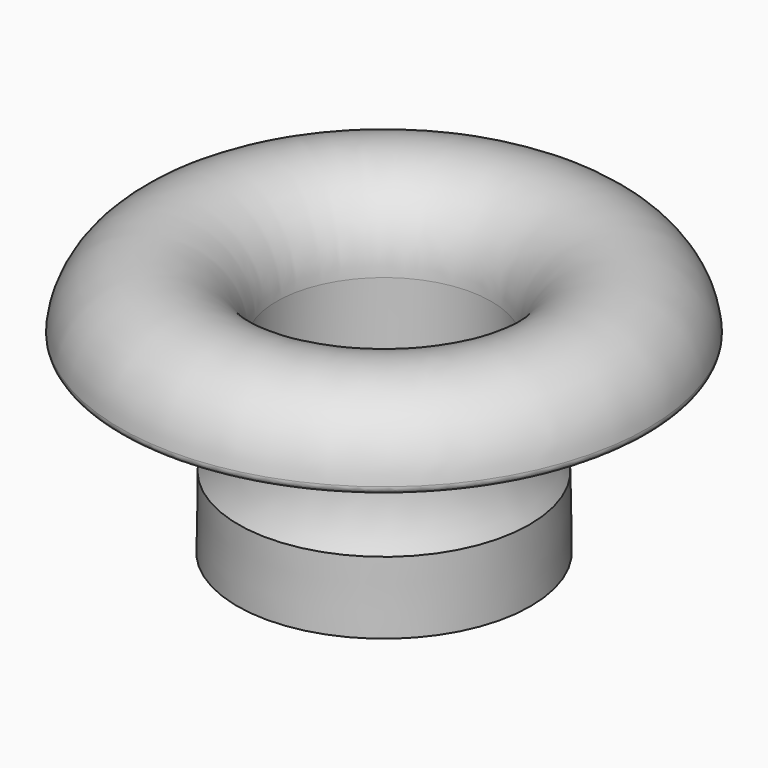
from build123d import *

# Parameters (mm, degrees)
F2_R    = 1
F3_SIZE = 1


# Not quite as in the source:
# - a feature names something its author has since deleted; it is built from what else it names


with BuildPart() as f1:
    # F0 (on Front) → F1 (revolve)
    with BuildSketch(Plane.XZ):
        with BuildLine():
            Line((18.9666396311, 19.1683829889), (21.9345718714, 19.1683829889))
            ThreePointArc((21.9345718714, 19.1683829889), (10.8824456559, 30.1359920722), (0, 19))
            Line((0, 19), (0, 3))
            Line((0, 3), (2.5, 3))
            Line((2.5, 3), (2.5, -7))
            Line((2.5, -7), (5.4997037066, -6.957837548))
            Line((5.4997037066, -6.957837548), (5.3591622, 3.0411748075))
            ThreePointArc((5.3591622, 3.0411748075), (3.5771962529, 6.9323566355), (2.9666396311, 11.1683829889))
            Line((2.9666396311, 11.1683829889), (2.9666396311, 19.1683829889))
            ThreePointArc((2.9666396311, 19.1683829889), (10.9666396311, 27.1683829889), (18.9666396311, 19.1683829889))
        make_face()
    revolve(axis=Axis((-15, 0, 28.4551028162), (0, 0, 1)))

    # F2
    f2_edges = [f1.edges().sort_by_distance(p)[0] for p in [
        (-51.934572, 0, 19.168383),
        (-48.96664, 0, 19.168383),
    ]]
    fillet(f2_edges, radius=F2_R)

    # F3
    f3_edges = [f1.edges().sort_by_distance(p)[0] for p in [
        (-32.5, 0, -7),
    ]]
    chamfer(f3_edges, length=F3_SIZE)


solid = f1.part
